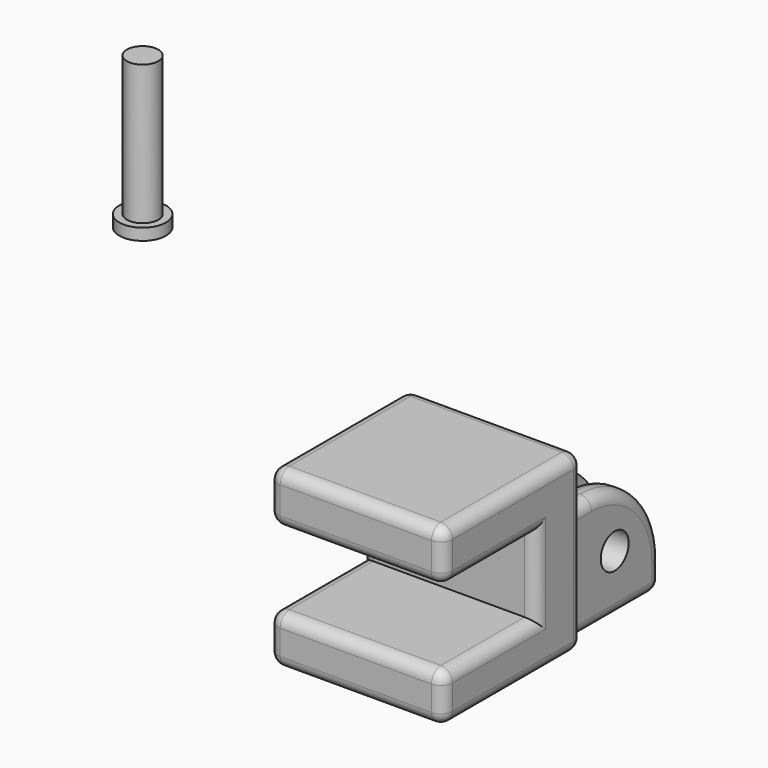
from build123d import *

# Parameters (mm, degrees)
F0_W       = 15
F0_H       = 15
F1_DEPTH   = 15
F2_W       = 15
F2_H       = 6.5
F1_FACE1_W = 15
F1_FACE1_H = 15
F3_DEPTH   = 10
F4_W       = 2.5
F4_H       = 10
F5_DEPTH   = 10
F6_R       = 1.5
F7_DEPTH   = 13.751
F8_R       = 7.5
F9_R       = 1
F0_R       = 1.35
F10_DEPTH  = 13
F0_R_2     = 2
F11_DEPTH  = 1


with BuildPart() as f1:
    # F0 (on Top) → F1 (new body)
    with BuildSketch(Plane.XY):
        Rectangle(F0_W, F0_H)
    extrude(amount=F1_DEPTH)

    # F2 (on face) + F1_face1 (on face) → F3 (cut)
    with BuildSketch(Plane.XZ.offset(7.5)):
        with Locations((0, 7.3964549899)):
            Rectangle(F2_W, F2_H)
    with BuildSketch(Plane(origin=(0, 7.5, 7.5), x_dir=(-1, 0, 0), z_dir=(0, 1, 0))):
        Rectangle(F1_FACE1_W, F1_FACE1_H)
    extrude(amount=-F3_DEPTH, dir=(0, -1, 0), mode=Mode.SUBTRACT)

    # F4 (on face) → F5 (join)
    with BuildSketch(Plane(origin=(0, 7.5, 0), x_dir=(-1, 0, 0), z_dir=(0, 1, 0))):
        with Locations((-5, 5)):
            Rectangle(F4_W, F4_H)
        with Locations((0, 5)):
            Rectangle(F4_W, F4_H)
        with Locations((5, 5)):
            Rectangle(F4_W, F4_H)
    extrude(amount=F5_DEPTH)

    # F6 (on face) → F7 (cut, through all)
    with BuildSketch(Plane.YZ.offset(6.25)):
        with Locations((12.5, 5)):
            Circle(F6_R)
    extrude(amount=-F7_DEPTH, mode=Mode.SUBTRACT)

    # F8
    f8_edges = [f1.edges().sort_by_distance(p)[0] for p in [
        (5, 17.5, 10),
        (0, 17.5, 10),
        (-5, 17.5, 10),
    ]]
    fillet(f8_edges, radius=F8_R)

    # F9
    f9_edges = [f1.edges().sort_by_distance(p)[0] for p in [
        (0, -7.5, 10.646455),
        (0, -7.5, 4.146455),
        (7.5, -2.5, 4.146455),
        (7.5, -2.5, 10.646455),
        (7.5, 0, 0),
        (7.5, 7.5, 7.5),
        (7.5, 0, 15),
        (7.5, -7.5, 12.823227),
        (7.5, 2.5, 7.396455),
        (7.5, -7.5, 2.073227),
        (-7.5, 0, 0),
        (-7.5, -7.5, 2.073227),
        (-7.5, -2.5, 4.146455),
        (-7.5, 2.5, 7.396455),
        (-7.5, -2.5, 10.646455),
        (-7.5, -7.5, 12.823227),
        (-7.5, 0, 15),
        (-7.5, 7.5, 7.5),
        (0, -7.5, 15),
        (0, 7.5, 15),
        (0, -7.5, 0),
        (6.875, 7.5, 0),
        (6.25, 12.5, 0),
        (5, 17.5, 0),
        (3.75, 12.5, 0),
        (2.5, 7.5, 0),
        (1.25, 12.5, 0),
        (0, 17.5, 0),
        (-1.25, 12.5, 0),
        (-2.5, 7.5, 0),
        (-3.75, 12.5, 0),
        (-5, 17.5, 0),
        (-6.25, 12.5, 0),
        (-6.875, 7.5, 0),
        (3.75, 15.303301, 7.803301),
        (5, 17.5, 2.5),
        (5, 10, 10),
        (6.25, 15.303301, 7.803301),
        (-1.25, 15.303301, 7.803301),
        (-6.25, 15.303301, 7.803301),
        (-5, 17.5, 2.5),
        (-5, 10, 10),
        (-3.75, 15.303301, 7.803301),
    ]]
    fillet(f9_edges, radius=F9_R)


with BuildPart() as f10:
    # F0 (on Top) → F10 (new body)
    with BuildSketch(Plane.XY):
        with Locations((-53.8979321718, 36.9674563408)):
            Circle(F0_R)
    extrude(amount=F10_DEPTH)

    # F0 (on Top) → F11 (join)
    with BuildSketch(Plane.XY):
        with Locations((-53.8979321718, 36.9674563408)):
            Circle(F0_R_2)
        with Locations((-53.8979321718, 36.9674563408)):
            Circle(F0_R, mode=Mode.SUBTRACT)
    extrude(amount=F11_DEPTH)


solid = Compound([f1.part, f10.part])
